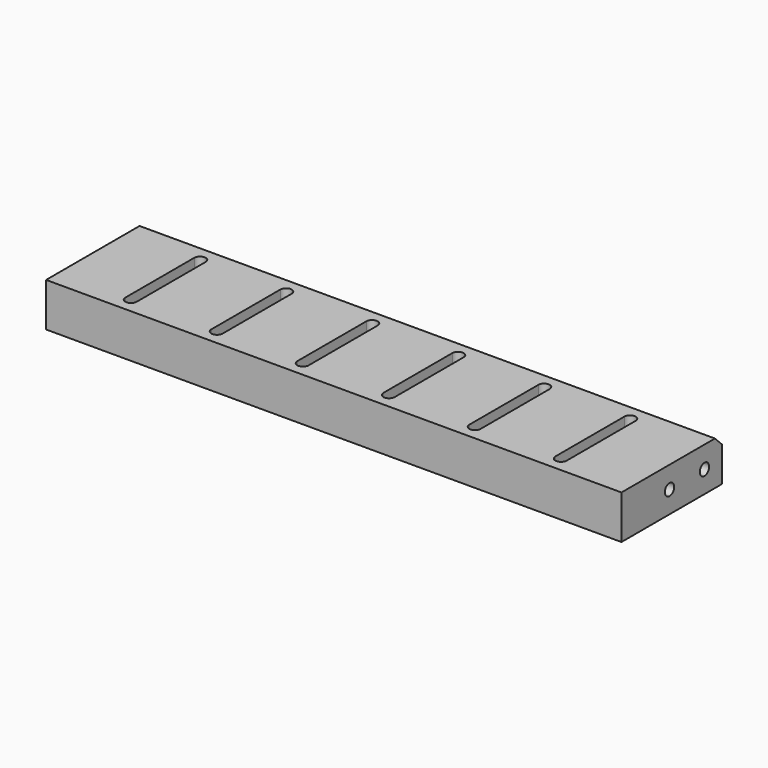
from build123d import *

# Parameters (mm, degrees)
F0_W      = 334.6
F0_H      = 73.025
F1_DEPTH  = 25.4
F2_SIZE   = 5.08
F4_D      = 6.8
F4_DEPTH  = 23.15
F4_TIP    = 2.0429261047
F6_D      = 6.8
F6_DEPTH  = 23.1394
F6_TIP    = 2.0429261047
F8_D      = 6.6
F10_DEPTH = 25.4
F12_DEPTH = 25.4


# Not quite as in the source:
# - a feature names something its author has since deleted; it is built from what else it names


with BuildPart() as f1:
    # F0 (on Top) → F1 (new body)
    with BuildSketch(Plane.XY):
        with Locations((164.5870582715, 36.5125)):
            Rectangle(F0_W, F0_H)
    extrude(amount=F1_DEPTH)

    # F2
    f2_edges = [f1.edges().sort_by_distance(p)[0] for p in [
        (164.587058, 73.025, 25.4),
    ]]
    chamfer(f2_edges, length=F2_SIZE)

    # F4
    with Locations(Plane.YZ.offset(331.8870582715)):
        with Locations((34.925, 12.7), (60.325, 12.7)):
            Hole(F4_D / 2, depth=F4_DEPTH)
            with Locations((0, 0, -(F4_DEPTH + F4_TIP / 2))):  # 118° drill point
                Cone(0, F4_D / 2, F4_TIP, mode=Mode.SUBTRACT)

    # F6
    with Locations(Plane(origin=(-2.7129417285, 0, 0), x_dir=(0, -1, 0), z_dir=(-1, 0, 0))):
        with Locations((-60.325, 12.7), (-34.925, 12.7)):
            Hole(F6_D / 2, depth=F6_DEPTH)
            with Locations((0, 0, -(F6_DEPTH + F6_TIP / 2))):  # 118° drill point
                Cone(0, F6_D / 2, F6_TIP, mode=Mode.SUBTRACT)

    # F8 (through all)
    with Locations(Plane.XY.offset(25.4)):
        with Locations((289.6185582715, 8.89), (289.6185582715, 59.055)):
            Hole(F8_D / 2)

    # F9 (on face) → F10 (cut)
    with BuildSketch(Plane.XY.offset(25.4)):
        with BuildLine():
            ThreePointArc((286.3185582715, 8.89), (289.6185582715, 12.19), (292.9185582715, 8.89))
            Line((292.9185582715, 8.89), (292.9185582715, 59.055))
            ThreePointArc((292.9185582715, 59.055), (289.6185582715, 55.755), (286.3185582715, 59.055))
            Line((286.3185582715, 59.055), (286.3185582715, 8.89))
        make_face()
    extrude(amount=-F10_DEPTH, mode=Mode.SUBTRACT)

    # F11 (on face) → F12 (cut)
    with BuildSketch(Plane.XY.offset(25.4)):
        with BuildLine():
            ThreePointArc((236.3059582715, 8.89), (239.6059582715, 5.59), (242.9059582715, 8.89))
            Line((242.9059582715, 8.89), (242.9059582715, 59.055))
            ThreePointArc((242.9059582715, 59.055), (239.6059582715, 62.355), (236.3059582715, 59.055))
            Line((236.3059582715, 59.055), (236.3059582715, 8.89))
        make_face()
        with BuildLine():
            ThreePointArc((186.2933582715, 8.89), (189.5933582715, 5.59), (192.8933582715, 8.89))
            Line((192.8933582715, 8.89), (192.8933582715, 59.055))
            ThreePointArc((192.8933582715, 59.055), (189.5933582715, 62.355), (186.2933582715, 59.055))
            Line((186.2933582715, 59.055), (186.2933582715, 8.89))
        make_face()
        with BuildLine():
            ThreePointArc((136.2807582715, 8.89), (139.5807582715, 5.59), (142.8807582715, 8.89))
            Line((142.8807582715, 8.89), (142.8807582715, 59.055))
            ThreePointArc((142.8807582715, 59.055), (139.5807582715, 62.355), (136.2807582715, 59.055))
            Line((136.2807582715, 59.055), (136.2807582715, 8.89))
        make_face()
        with BuildLine():
            ThreePointArc((86.2681582715, 8.89), (89.5681582715, 5.59), (92.8681582715, 8.89))
            Line((92.8681582715, 8.89), (92.8681582715, 59.055))
            ThreePointArc((92.8681582715, 59.055), (89.5681582715, 62.355), (86.2681582715, 59.055))
            Line((86.2681582715, 59.055), (86.2681582715, 8.89))
        make_face()
        with BuildLine():
            ThreePointArc((36.2555582715, 8.89), (39.5555582715, 5.59), (42.8555582715, 8.89))
            Line((42.8555582715, 8.89), (42.8555582715, 59.055))
            ThreePointArc((42.8555582715, 59.055), (39.5555582715, 62.355), (36.2555582715, 59.055))
            Line((36.2555582715, 59.055), (36.2555582715, 8.89))
        make_face()
    extrude(amount=-F12_DEPTH, mode=Mode.SUBTRACT)


solid = f1.part
